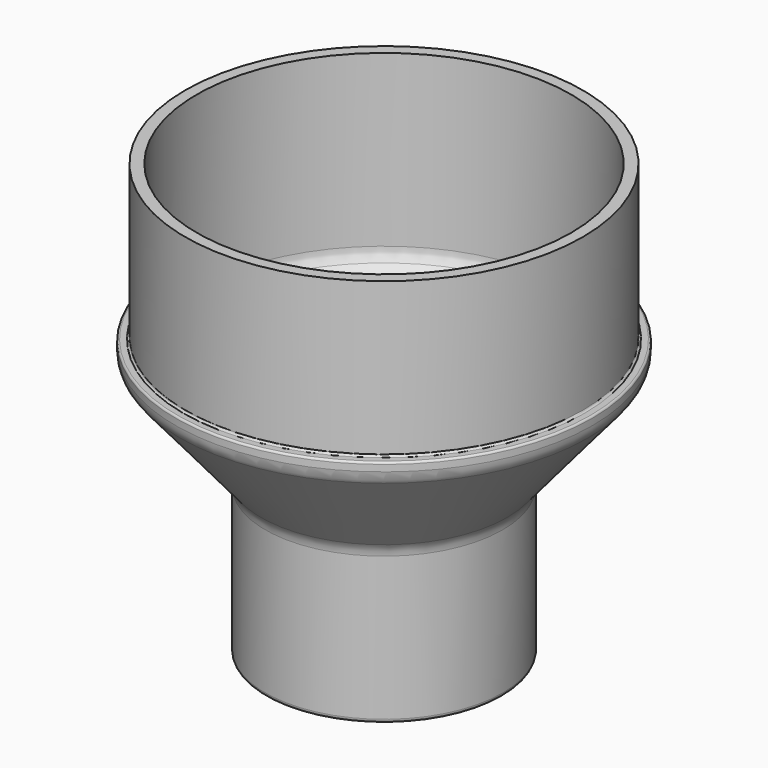
from build123d import *

# Parameters (mm, degrees)
F2_R = 0.5
F3_R = 1


# Not quite as in the source:
# - a feature names something its author has since deleted; it is built from what else it names


with BuildPart() as f1:
    # F0 (on Front) → F1 (revolve)
    with BuildSketch(Plane.XZ):
        with BuildLine():
            Line((27.75, 0), (30.75, 0))
            Line((30.75, 0), (30.75, 38.1801488287))
            ThreePointArc((30.75, 38.1801488287), (31.0515368961, 39.8902495453), (31.9197777844, 41.3940868771))
            Line((31.9197777844, 41.3940868771), (52.8302222156, 66.3141841507))
            ThreePointArc((52.8302222156, 66.3141841507), (53.6984631039, 67.8180214825), (54, 69.5281221991))
            Line((54, 69.5281221991), (54, 71.7082710278))
            Line((54, 71.7082710278), (51.5, 71.7082710278))
            Line((51.5, 71.7082710278), (51.5, 111.7082710278))
            Line((51.5, 111.7082710278), (48.5, 111.7082710278))
            Line((48.5, 111.7082710278), (48.5, 67.6406489205))
            ThreePointArc((48.5, 67.6406489205), (48.1984631039, 65.9305482038), (47.3302222156, 64.426710872))
            Line((47.3302222156, 64.426710872), (28.9197777844, 42.4859975799))
            ThreePointArc((28.9197777844, 42.4859975799), (28.0515368961, 40.9821602481), (27.75, 39.2720595315))
            Line((27.75, 39.2720595315), (27.75, 0))
        make_face()
    revolve(axis=Axis((0, 0, 46.6845482588), (0, 0, 1)))

    # F2
    f2_edges = [f1.edges().sort_by_distance(p)[0] for p in [
        (-54, 0, 71.708271),
        (-51.5, 0, 71.708271),
    ]]
    fillet(f2_edges, radius=F2_R)

    # F3
    f3_edges = [f1.edges().sort_by_distance(p)[0] for p in [
        (-30.75, 0, 0),
        (-27.75, 0, 0),
    ]]
    fillet(f3_edges, radius=F3_R)


solid = f1.part
